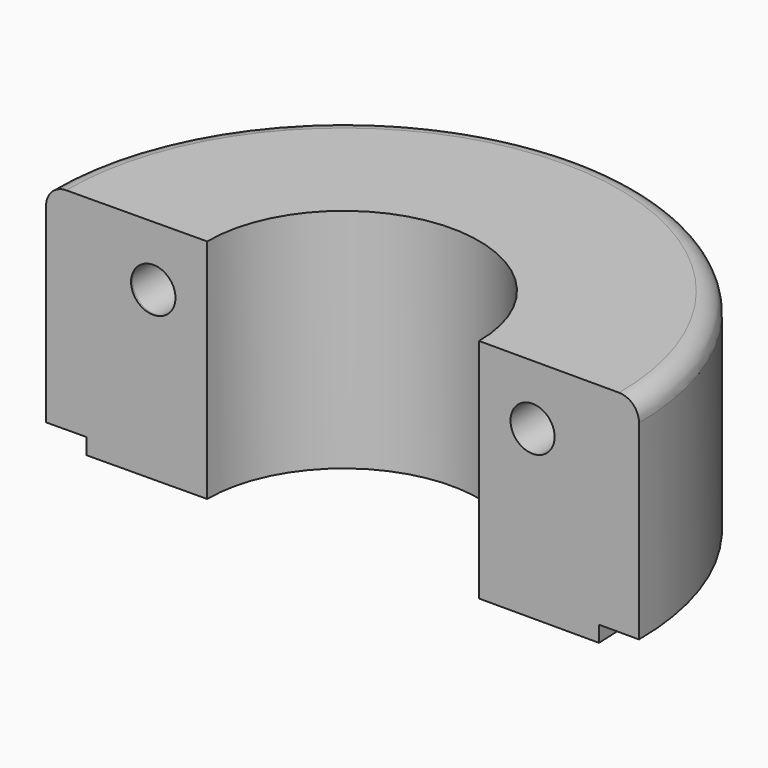
from build123d import *

# Parameters (mm, degrees)
F1_ANGLE_BACK = 180.5
F1_ANGLE      = 180.5
F2_R          = 3.5
F3_DEPTH      = 53.34
F3_DEPTH_BACK = 2.54
F6_DEPTH      = 35.56


# Not quite as in the source:
# - a feature names something its author has since deleted; it is built from what else it names


with BuildPart() as f1:
    # F0 (on Front) → F1 (revolve)
    with BuildSketch(Plane.XZ, mode=Mode.PRIVATE) as f1_sk:
        with BuildLine():
            Line((21.5, 36), (21.5, 0))
            Line((21.5, 0), (40.55, 0))
            Line((40.55, 0), (40.55, 2.54))
            Line((40.55, 2.54), (46.9, 2.54))
            Line((46.9, 2.54), (46.9, 32.825))
            ThreePointArc((46.9, 32.825), (45.9700640303, 35.0700640303), (43.725, 36))
            Line((43.725, 36), (21.5, 36))
        make_face()
    revolve(f1_sk.sketch.rotate(Axis((0, 0, -0.0018208164), (0, 0, -1)), -F1_ANGLE_BACK), axis=Axis((0, 0, -0.0018208164), (0, 0, -1)), revolution_arc=F1_ANGLE)

    # F2 (on Front) → F3 (cut, two sides)
    with BuildSketch(Plane.XZ) as f3_sk:
        with Locations((30, 26.5004)):
            Circle(F2_R)
        with Locations((-30, 26.5004)):
            Circle(F2_R)
    extrude(amount=-F3_DEPTH, mode=Mode.SUBTRACT)
    extrude(f3_sk.sketch, amount=F3_DEPTH_BACK, mode=Mode.SUBTRACT)

    # F5 (on offset) → F6 (cut)
    with BuildSketch(Plane.XZ.offset(-50.8)):
        Polygon((36.6991664547, 26.5004), (33.3482832273, 32.3043), (26.6465167727, 32.3043), (23.2956335453, 26.5004), (26.6465167727, 20.6965), (33.3482832273, 20.6965), align=None)
        Polygon((-33.3482832273, 32.3043), (-36.6991664547, 26.5004), (-33.3482832273, 20.6965), (-26.6465167727, 20.6965), (-23.2956335453, 26.5004), (-26.6465167727, 32.3043), align=None)
    extrude(amount=F6_DEPTH, mode=Mode.SUBTRACT)


solid = f1.part
